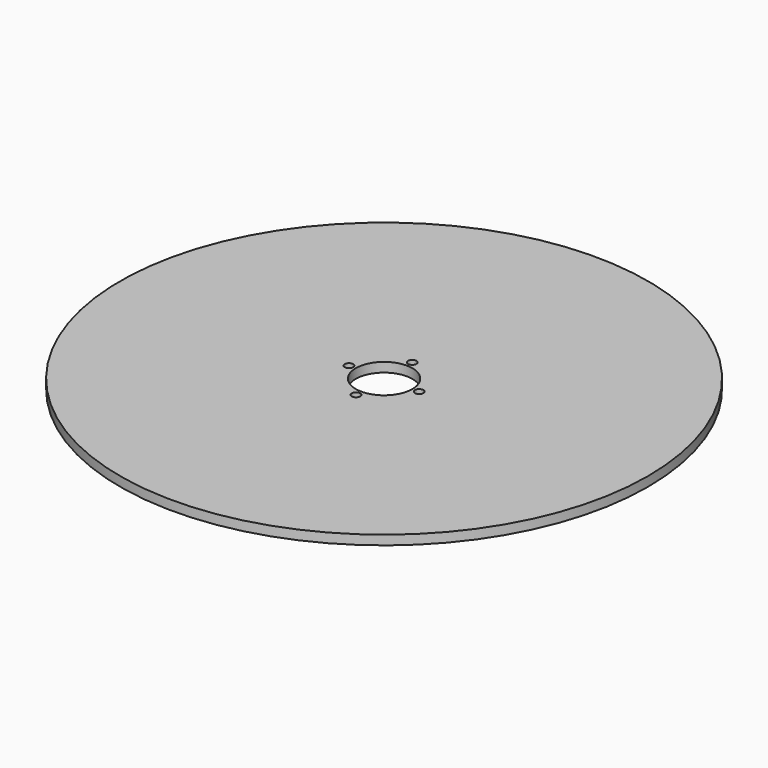
from build123d import *

# Parameters (mm, degrees)
F0_R     = 280
F1_DEPTH = 10
F2_R     = 30
F2_R_2   = 4.5
F3_DEPTH = 25


# Not quite as in the source:
# - a feature names something its author has since deleted; it is built from what else it names


with BuildPart() as f1:
    # F0 (on Top) → F1 (new body)
    with BuildSketch(Plane.XY):
        Circle(F0_R)
    extrude(amount=F1_DEPTH)

    # F2 (on face) → F3 (cut)
    with BuildSketch(Plane.XY.offset(10)):
        Circle(F2_R)
        with Locations((-37.25, 0)):
            Circle(F2_R_2)
        with Locations((0, 37.25)):
            Circle(F2_R_2)
        with Locations((37.25, 0)):
            Circle(F2_R_2)
        with Locations((0, -37.25)):
            Circle(F2_R_2)
    extrude(amount=-F3_DEPTH, mode=Mode.SUBTRACT)


solid = f1.part
